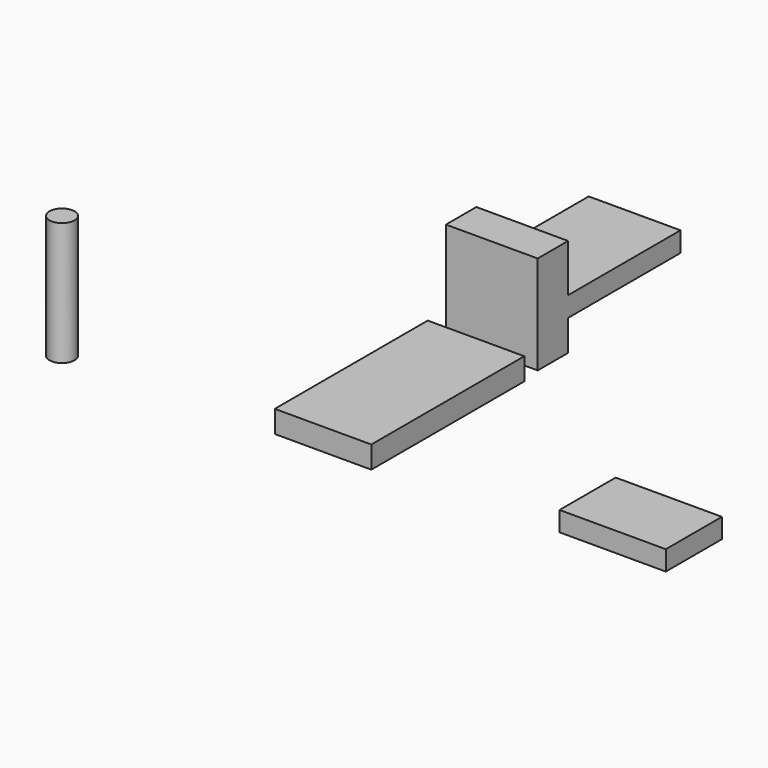
from build123d import *

# Parameters (mm, degrees)
F2_W      = 39.1845554113
F2_H      = 77.5835588574
F3_DEPTH  = 9
F4_W      = 37.2421750799
F4_H      = 15.4253318906
F5_DEPTH  = 40
F6_W      = 37.2421750799
F6_H      = 8.1134717911
F7_DEPTH  = 16
F8_DEPTH  = 25
F9_DEPTH  = 15
F10_DEPTH = 1
F11_DEPTH = 20
F12_R     = 5.0490195459
F13_DEPTH = 50
F14_W     = 43.1157648563
F14_H     = 28.46735809
F15_DEPTH = 8


# Not quite as in the source:
# - the program builds the solid bodies; features that only make, move or delete a surface that nothing else refers to are left out


with BuildPart() as f3:
    # F2 (on Top) → F3 (new body)
    with BuildSketch(Plane.XY):
        with Locations((8.1322155893, -4.6339258552)):
            Rectangle(F2_W, F2_H)
    extrude(amount=F3_DEPTH)


with BuildPart() as f5:
    # F4 (on Top) → F5 (new body)
    with BuildSketch(Plane.XY):
        with Locations((7.7287382446, 50.4066199064)):
            Rectangle(F4_W, F4_H)
    extrude(amount=F5_DEPTH)

    # F6 (on face) → F7 (join)
    with BuildSketch(Plane(origin=(0, 58.1192858517, 0), x_dir=(-1, 0, 0), z_dir=(0, 1, 0))):
        with Locations((-7.7287382446, 16.5685703978)):
            Rectangle(F6_W, F6_H)
    extrude(amount=F7_DEPTH)

    # F8 (add): a face of the model
    f8_faces = [f5.faces().sort_by_distance(p)[0] for p in [
        (7.7287382446, 74.1192858517, 16.5685703978),
    ]]
    extrude(f8_faces, amount=F8_DEPTH)

    # F9 (add): a face of the model
    f9_faces = [f5.faces().sort_by_distance(p)[0] for p in [
        (7.7287382446, 99.1192858517, 16.5685703978),
    ]]
    extrude(f9_faces, amount=F9_DEPTH)

    # F10 (add): a face of the model
    f10_faces = [f5.faces().sort_by_distance(p)[0] for p in [
        (7.7287382446, 114.1192858517, 16.5685703978),
    ]]
    extrude(f10_faces, amount=F10_DEPTH)

    # F11 (add): a face of the model
    f11_faces = [f5.faces().sort_by_distance(p)[0] for p in [
        (7.7287382446, 115.1192858517, 16.5685703978),
    ]]
    extrude(f11_faces, amount=-F11_DEPTH)


with BuildPart() as f13:
    # F12 (on Top) → F13 (new body)
    with BuildSketch(Plane.XY):
        with Locations((-97.6576507092, -43.5994267464)):
            Circle(F12_R)
    extrude(amount=F13_DEPTH)


with BuildPart() as f15:
    # F14 (on Top) → F15 (new body)
    with BuildSketch(Plane.XY):
        with Locations((122.7215528488, -25.5093905143)):
            Rectangle(F14_W, F14_H)
    extrude(amount=F15_DEPTH)


solid = Compound([f3.part, f5.part, f13.part, f15.part])
